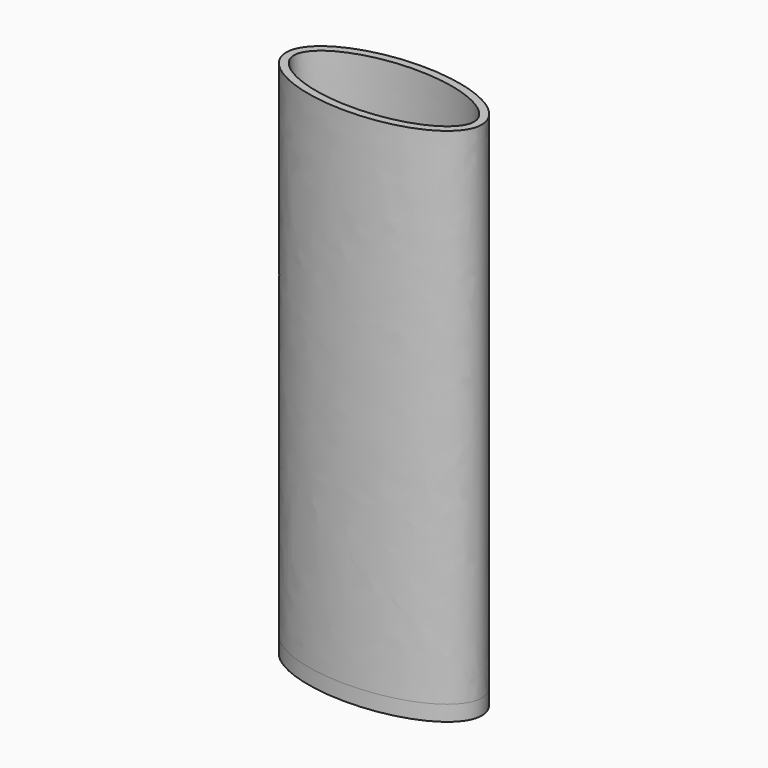
from build123d import *

# Parameters (mm, degrees)
F1_DEPTH = 65
F2_DEPTH = 2


# Not quite as in the source:
# - the dataset's text gives a spline's control points without its knots; the knots are read off the source's solid


with BuildPart() as f1:
    # F0 (on Top) → F1 (new body)
    with BuildSketch(Plane.XY):
        with BuildLine():
            add(Edge.make_bspline(
                [(12.6, 0), (12.6, 10.7387150069), (-6.3, 5.3693575035), (-25.2, 0), (-6.3, -5.3693575035), (12.6, -10.7387150069), (12.6, 0)],
                knots=[0, 0, 0, 2.0943951024, 2.0943951024, 4.1887902048, 4.1887902048, 6.2831853072, 6.2831853072, 6.2831853072], degree=2, weights=[1, 0.5, 1, 0.5, 1, 0.5, 1]))
        make_face()
        with BuildLine():
            add(Edge.make_bspline(
                [(11.6, 0), (11.6, 0.2742138603), (11.4943541756, 0.8226415809), (11.0428725229, 1.5725942573), (10.454737187, 2.1868891174), (9.7142468376, 2.795917269), (8.5286217571, 3.5086701034), (7.0400300216, 4.1120721714), (5.6929691733, 4.5095892166), (4.2711535866, 4.8402086313), (2.7584453229, 5.0660415884), (1.1932120753, 5.1806364813), (0, 5.2096817593), (-1.1932120753, 5.1806364813), (-2.7584453229, 5.0660415884), (-4.2711535866, 4.8402086313), (-5.6929691733, 4.5095892166), (-7.0400300216, 4.1120721714), (-8.5286217571, 3.5086701034), (-9.7142468376, 2.795917269), (-10.454737187, 2.1868891174), (-11.0428725229, 1.5725942573), (-11.4943541756, 0.8226415809), (-11.6528229122, 0), (-11.4943541756, -0.8226415809), (-11.0428725229, -1.5725942573), (-10.454737187, -2.1868891174), (-9.7142468376, -2.795917269), (-8.5286217571, -3.5086701034), (-7.0400300216, -4.1120721714), (-5.6929691733, -4.5095892166), (-4.2711535866, -4.8402086313), (-2.7584453229, -5.0660415884), (-1.1932120753, -5.1806364813), (0, -5.2096817593), (1.1932120753, -5.1806364813), (2.7584453229, -5.0660415884), (4.2711535866, -4.8402086313), (5.6929691733, -4.5095892166), (7.0400300216, -4.1120721714), (8.5286217571, -3.5086701034), (9.7142468376, -2.795917269), (10.454737187, -2.1868891174), (11.0428725229, -1.5725942573), (11.4943541756, -0.8226415809), (11.6, -0.2742138603), (11.6, 0)],
                knots=[0, 0, 0, 0, 0.03125, 0.0625, 0.078125, 0.09375, 0.125, 0.15625, 0.171875, 0.1875, 0.21875, 0.234375, 0.25, 0.265625, 0.28125, 0.3125, 0.328125, 0.34375, 0.375, 0.40625, 0.421875, 0.4375, 0.46875, 0.5, 0.53125, 0.5625, 0.578125, 0.59375, 0.625, 0.65625, 0.671875, 0.6875, 0.71875, 0.734375, 0.75, 0.765625, 0.78125, 0.8125, 0.828125, 0.84375, 0.875, 0.90625, 0.921875, 0.9375, 0.96875, 1, 1, 1, 1], degree=3))
        make_face(mode=Mode.SUBTRACT)
    extrude(amount=F1_DEPTH)

    # F1_face (on face) + F0 (on Top) → F2 (join)
    with BuildSketch(Plane(origin=(0.2988225551, 0, 0), x_dir=(1, 0, 0), z_dir=(0, 0, -1))):
        with BuildLine():
            add(Edge.make_bspline(
                [(12.3011774449, 0), (12.3011774449, -10.7387150069), (-6.5988225551, -5.3693575035), (-25.4988225551, 0), (-6.5988225551, 5.3693575035), (12.3011774449, 10.7387150069), (12.3011774449, 0)],
                knots=[0, 0, 0, 2.0943951024, 2.0943951024, 4.1887902048, 4.1887902048, 6.2831853072, 6.2831853072, 6.2831853072], degree=2, weights=[1, 0.5, 1, 0.5, 1, 0.5, 1]))
        make_face()
        with BuildLine():
            add(Edge.make_bspline(
                [(11.3011774449, 0), (11.3011774449, -0.2742138603), (11.1955316205, -0.8226415809), (10.7440499678, -1.5725942573), (10.1559146319, -2.1868891174), (9.4154242825, -2.795917269), (8.229799202, -3.5086701034), (6.7412074664, -4.1120721714), (5.3941466182, -4.5095892166), (3.9723310315, -4.8402086313), (2.4596227678, -5.0660415884), (0.8943895202, -5.1806364813), (-0.2988225551, -5.2096817593), (-1.4920346304, -5.1806364813), (-3.057267878, -5.0660415884), (-4.5699761417, -4.8402086313), (-5.9917917284, -4.5095892166), (-7.3388525767, -4.1120721714), (-8.8274443123, -3.5086701034), (-10.0130693927, -2.795917269), (-10.7535597421, -2.1868891174), (-11.341695078, -1.5725942573), (-11.7931767308, -0.8226415809), (-11.9516454673, 0), (-11.7931767308, 0.8226415809), (-11.341695078, 1.5725942573), (-10.7535597421, 2.1868891174), (-10.0130693927, 2.795917269), (-8.8274443123, 3.5086701034), (-7.3388525767, 4.1120721714), (-5.9917917284, 4.5095892166), (-4.5699761417, 4.8402086313), (-3.057267878, 5.0660415884), (-1.4920346304, 5.1806364813), (-0.2988225551, 5.2096817593), (0.8943895202, 5.1806364813), (2.4596227678, 5.0660415884), (3.9723310315, 4.8402086313), (5.3941466182, 4.5095892166), (6.7412074664, 4.1120721714), (8.229799202, 3.5086701034), (9.4154242825, 2.795917269), (10.1559146319, 2.1868891174), (10.7440499678, 1.5725942573), (11.1955316205, 0.8226415809), (11.3011774449, 0.2742138603), (11.3011774449, 0)],
                knots=[0, 0, 0, 0, 0.03125, 0.0625, 0.078125, 0.09375, 0.125, 0.15625, 0.171875, 0.1875, 0.21875, 0.234375, 0.25, 0.265625, 0.28125, 0.3125, 0.328125, 0.34375, 0.375, 0.40625, 0.421875, 0.4375, 0.46875, 0.5, 0.53125, 0.5625, 0.578125, 0.59375, 0.625, 0.65625, 0.671875, 0.6875, 0.71875, 0.734375, 0.75, 0.765625, 0.78125, 0.8125, 0.828125, 0.84375, 0.875, 0.90625, 0.921875, 0.9375, 0.96875, 1, 1, 1, 1], degree=3))
        make_face(mode=Mode.SUBTRACT)
    with BuildSketch(Plane.XY):
        with BuildLine():
            add(Edge.make_bspline(
                [(12.6, 0), (12.6, 10.7387150069), (-6.3, 5.3693575035), (-25.2, 0), (-6.3, -5.3693575035), (12.6, -10.7387150069), (12.6, 0)],
                knots=[0, 0, 0, 2.0943951024, 2.0943951024, 4.1887902048, 4.1887902048, 6.2831853072, 6.2831853072, 6.2831853072], degree=2, weights=[1, 0.5, 1, 0.5, 1, 0.5, 1]))
        make_face()
        with BuildLine():
            add(Edge.make_bspline(
                [(11.6, 0), (11.6, 0.2742138603), (11.4943541756, 0.8226415809), (11.0428725229, 1.5725942573), (10.454737187, 2.1868891174), (9.7142468376, 2.795917269), (8.5286217571, 3.5086701034), (7.0400300216, 4.1120721714), (5.6929691733, 4.5095892166), (4.2711535866, 4.8402086313), (2.7584453229, 5.0660415884), (1.1932120753, 5.1806364813), (0, 5.2096817593), (-1.1932120753, 5.1806364813), (-2.7584453229, 5.0660415884), (-4.2711535866, 4.8402086313), (-5.6929691733, 4.5095892166), (-7.0400300216, 4.1120721714), (-8.5286217571, 3.5086701034), (-9.7142468376, 2.795917269), (-10.454737187, 2.1868891174), (-11.0428725229, 1.5725942573), (-11.4943541756, 0.8226415809), (-11.6528229122, 0), (-11.4943541756, -0.8226415809), (-11.0428725229, -1.5725942573), (-10.454737187, -2.1868891174), (-9.7142468376, -2.795917269), (-8.5286217571, -3.5086701034), (-7.0400300216, -4.1120721714), (-5.6929691733, -4.5095892166), (-4.2711535866, -4.8402086313), (-2.7584453229, -5.0660415884), (-1.1932120753, -5.1806364813), (0, -5.2096817593), (1.1932120753, -5.1806364813), (2.7584453229, -5.0660415884), (4.2711535866, -4.8402086313), (5.6929691733, -4.5095892166), (7.0400300216, -4.1120721714), (8.5286217571, -3.5086701034), (9.7142468376, -2.795917269), (10.454737187, -2.1868891174), (11.0428725229, -1.5725942573), (11.4943541756, -0.8226415809), (11.6, -0.2742138603), (11.6, 0)],
                knots=[0, 0, 0, 0, 0.03125, 0.0625, 0.078125, 0.09375, 0.125, 0.15625, 0.171875, 0.1875, 0.21875, 0.234375, 0.25, 0.265625, 0.28125, 0.3125, 0.328125, 0.34375, 0.375, 0.40625, 0.421875, 0.4375, 0.46875, 0.5, 0.53125, 0.5625, 0.578125, 0.59375, 0.625, 0.65625, 0.671875, 0.6875, 0.71875, 0.734375, 0.75, 0.765625, 0.78125, 0.8125, 0.828125, 0.84375, 0.875, 0.90625, 0.921875, 0.9375, 0.96875, 1, 1, 1, 1], degree=3))
        make_face(mode=Mode.SUBTRACT)
        with BuildLine():
            add(Edge.make_bspline(
                [(11.6, 0), (11.6, 0.2742138603), (11.4943541756, 0.8226415809), (11.0428725229, 1.5725942573), (10.454737187, 2.1868891174), (9.7142468376, 2.795917269), (8.5286217571, 3.5086701034), (7.0400300216, 4.1120721714), (5.6929691733, 4.5095892166), (4.2711535866, 4.8402086313), (2.7584453229, 5.0660415884), (1.1932120753, 5.1806364813), (0, 5.2096817593), (-1.1932120753, 5.1806364813), (-2.7584453229, 5.0660415884), (-4.2711535866, 4.8402086313), (-5.6929691733, 4.5095892166), (-7.0400300216, 4.1120721714), (-8.5286217571, 3.5086701034), (-9.7142468376, 2.795917269), (-10.454737187, 2.1868891174), (-11.0428725229, 1.5725942573), (-11.4943541756, 0.8226415809), (-11.6528229122, 0), (-11.4943541756, -0.8226415809), (-11.0428725229, -1.5725942573), (-10.454737187, -2.1868891174), (-9.7142468376, -2.795917269), (-8.5286217571, -3.5086701034), (-7.0400300216, -4.1120721714), (-5.6929691733, -4.5095892166), (-4.2711535866, -4.8402086313), (-2.7584453229, -5.0660415884), (-1.1932120753, -5.1806364813), (0, -5.2096817593), (1.1932120753, -5.1806364813), (2.7584453229, -5.0660415884), (4.2711535866, -4.8402086313), (5.6929691733, -4.5095892166), (7.0400300216, -4.1120721714), (8.5286217571, -3.5086701034), (9.7142468376, -2.795917269), (10.454737187, -2.1868891174), (11.0428725229, -1.5725942573), (11.4943541756, -0.8226415809), (11.6, -0.2742138603), (11.6, 0)],
                knots=[0, 0, 0, 0, 0.03125, 0.0625, 0.078125, 0.09375, 0.125, 0.15625, 0.171875, 0.1875, 0.21875, 0.234375, 0.25, 0.265625, 0.28125, 0.3125, 0.328125, 0.34375, 0.375, 0.40625, 0.421875, 0.4375, 0.46875, 0.5, 0.53125, 0.5625, 0.578125, 0.59375, 0.625, 0.65625, 0.671875, 0.6875, 0.71875, 0.734375, 0.75, 0.765625, 0.78125, 0.8125, 0.828125, 0.84375, 0.875, 0.90625, 0.921875, 0.9375, 0.96875, 1, 1, 1, 1], degree=3))
        make_face()
    extrude(amount=F2_DEPTH, dir=(0, 0, -1))


solid = f1.part
